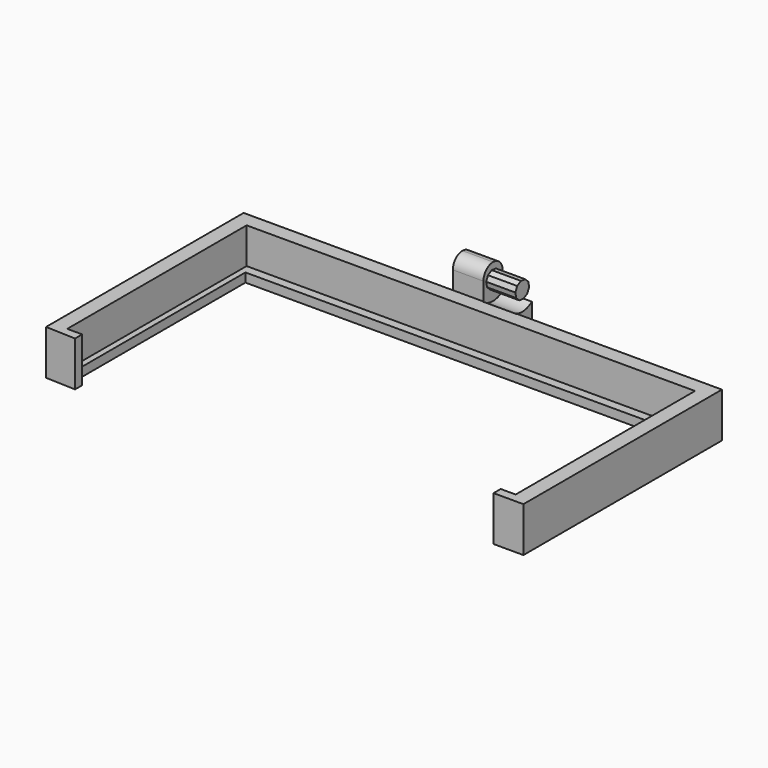
from build123d import *

# Parameters (mm, degrees)
F1_DEPTH = 15
F2_DEPTH = 3
F0_W     = 146
F0_H     = 3
F3_DEPTH = 3
F0_W_2   = 20
F0_H_2   = 8
F4_DEPTH = 25
F5_R     = 6.5
F6_DEPTH = 11.3693
F7_R     = 3.99999


# Not quite as in the source:
# - a fillet or chamfer is up to 0.001 mm smaller than in the source, because OpenCascade refuses the exact size


with BuildPart() as f1:
    # F0 (on Top) → F1 (new body)
    with BuildSketch(Plane.XY):
        Polygon((-21.6026537657, 32.1407727134), (-91.6026537657, 32.1407727134), (-91.6026537657, -50.4549115884), (-81.6026537657, -50.8592272866), (-81.6026537657, -47.8592272866), (-84.6026537657, -47.8592272866), (-86.6026537657, -47.8592272866), (-86.6026537657, 27.1407727134), (-84.6026537657, 27.1407727134), (61.3973462343, 27.1407727134), (63.3973462343, 27.1407727134), (63.3973462343, -47.8592272866), (61.3973462343, -47.8592272866), (58.3973462343, -47.8592272866), (58.3973462343, -50.8592272866), (68.3973462343, -50.8592272866), (68.3973462343, 32.1407727134), (-1.6026537657, 32.1407727134), align=None)
    extrude(amount=F1_DEPTH)

    # F0 (on Top) → F2 (join)
    with BuildSketch(Plane.XY):
        Polygon((-86.6026537657, -47.8592272866), (-84.6026537657, -47.8592272866), (-84.6026537657, 24.1407727134), (-84.6026537657, 27.1407727134), (-86.6026537657, 27.1407727134), align=None)
        Polygon((61.3973462343, 27.1407727134), (61.3973462343, 24.1407727134), (61.3973462343, -47.8592272866), (63.3973462343, -47.8592272866), (63.3973462343, 27.1407727134), align=None)
    extrude(amount=F2_DEPTH)

    # F0 (on Top) → F3 (join)
    with BuildSketch(Plane.XY):
        with Locations((-11.6026537657, 25.6407727134)):
            Rectangle(F0_W, F0_H)
    extrude(amount=F3_DEPTH)

    # F0 (on Top) → F4 (join)
    with BuildSketch(Plane.XY):
        with Locations((-11.6026537657, 36.1407727134)):
            Rectangle(F0_W_2, F0_H_2)
    extrude(amount=F4_DEPTH)

    # F5 (on Right) → F6 (cut)
    with BuildSketch(Plane.YZ):
        with Locations((36.1407727134, 20)):
            Circle(F5_R)
        Polygon((33.2721245414, 20.362976629), (34.0333399009, 21.979803351), (35.5995229657, 22.8404124839), (37.3724450378, 22.61608059), (38.674910145, 21.3924948281), (39.0094208855, 19.637023371), (38.248205526, 18.020196649), (36.6820224612, 17.1595875161), (34.9091003891, 17.38391941), (33.6066352819, 18.6075051719), align=None, mode=Mode.SUBTRACT)
    extrude(amount=-F6_DEPTH, mode=Mode.SUBTRACT)

    # F7 (radius 4 in the source; OpenCascade refuses exactly that, so slightly less here)
    f7_edges = [f1.edges().sort_by_distance(p)[0] for p in [
        (-16.485977, 40.140773, 25),
        (-16.485977, 32.140773, 25),
    ]]
    fillet(f7_edges, radius=F7_R)


solid = f1.part
